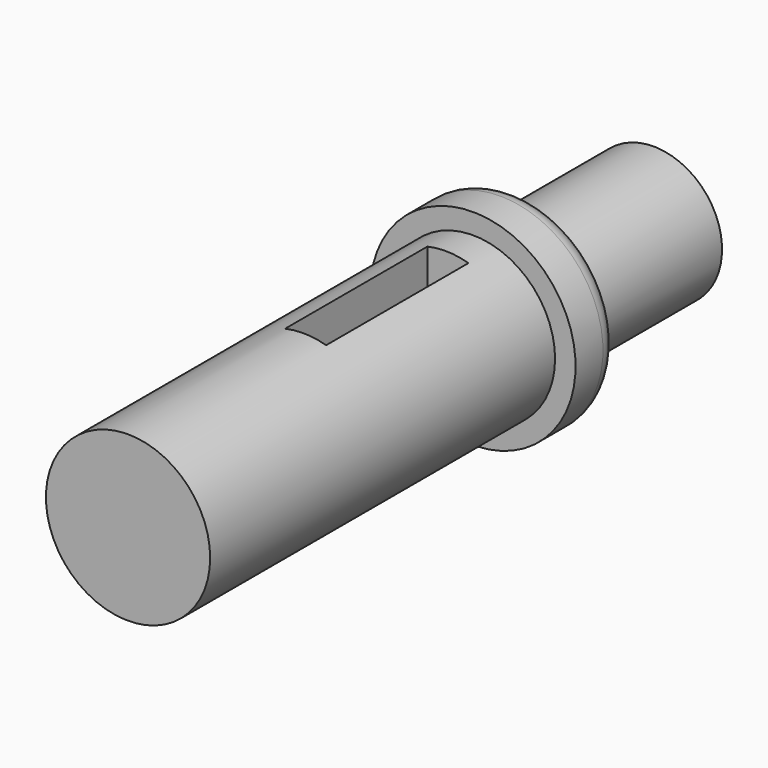
from build123d import *

# Parameters (mm, degrees)
F0_R     = 12
F1_DEPTH = 63
F2_R     = 15
F2_R_2   = 12
F3_DEPTH = 8
F4_R     = 10
F5_DEPTH = 25
F6_R     = 3
F8_DEPTH = 31.2849479744


with BuildPart() as f1:
    # F0 (on Front) → F1 (new body)
    with BuildSketch(Plane.XZ):
        with Locations((18.5694117099, 16.2839479744)):
            Circle(F0_R)
    extrude(amount=F1_DEPTH)

    # F2 (on face) → F3 (join)
    with BuildSketch(Plane(origin=(0, 0, 0), x_dir=(-1, 0, 0), z_dir=(0, 1, 0))):
        with Locations((-18.5694117099, 16.2839479744)):
            Circle(F2_R)
        with Locations((-18.5694117099, 16.2839479744)):
            Circle(F2_R_2, mode=Mode.SUBTRACT)
        with Locations((-18.5694117099, 16.2839479744)):
            Circle(F2_R_2)
    extrude(amount=F3_DEPTH)

    # F4 (on face) → F5 (join)
    with BuildSketch(Plane(origin=(0, 8, 0), x_dir=(-1, 0, 0), z_dir=(0, 1, 0))):
        with Locations((-18.5694117099, 16.2839479744)):
            Circle(F4_R)
    extrude(amount=F5_DEPTH)

    # F6
    f6_edges = [f1.edges().sort_by_distance(p)[0] for p in [
        (33.569412, 8, 16.283948),
    ]]
    fillet(f6_edges, radius=F6_R)

    # F7 (on Top) → F8 (cut, through all)
    with BuildSketch(Plane.XY):
        Polygon((21.912544474, -4.9977113605), (18.912544474, -4.9977113605), (15.912544474, -4.9977113605), (15.912544474, -30.9977113605), (18.912544474, -30.9977113605), (21.912544474, -30.9977113605), align=None)
    extrude(amount=F8_DEPTH, mode=Mode.SUBTRACT)


solid = f1.part
